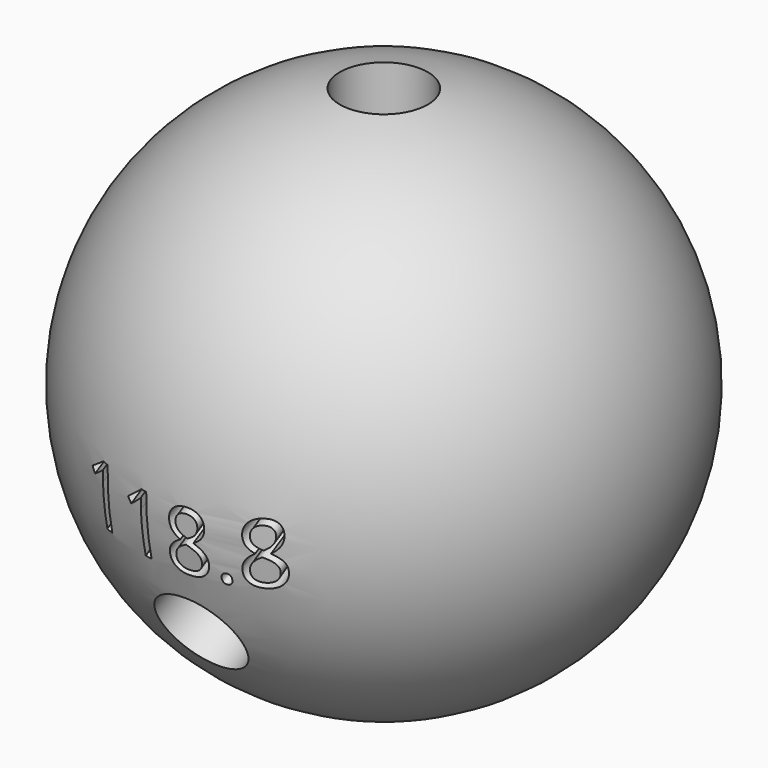
from build123d import *

# Parameters (mm, degrees)
F5_R          = 3.175
F6_DEPTH      = 76.2
F7_ANGLE      = 118.8
F8_ANGLE      = 119.3
F10_TEXT_SIZE = 5.7784387738
F11_DEPTH     = 6.35
F13_TEXT_SIZE = 6.645384969
F14_DEPTH     = 6.35


# Not quite as in the source:
# - Text() gives the source's letters only with a copy of the font that has no kerning and outlines rounded to 1/6400 em; it was checked with that copy


with BuildPart() as f2:
    # F0 (on Front) → F2 (revolve)
    with BuildSketch(Plane.XZ):
        with BuildLine():
            Line((0, -19.05), (0, 19.05))
            ThreePointArc((0, 19.05), (-19.05, 0), (0, -19.05))
        make_face()
    revolve(axis=Axis((0, 0, 0), (0, 0, 1)))

    # F10 (on offset) → F11 (cut)
    with BuildSketch(Plane(origin=(0, -17.8065517385, -9.7892346577), x_dir=(1, 0, 0), z_dir=(0, -0.87630668, -0.4817536741))):
        with Locations((-7.3158596642, 5.1700836048)):
            Text('118.8', F10_TEXT_SIZE, font='Open Sans', text_align=(TextAlign.LEFT, TextAlign.BOTTOM))
    extrude(amount=-F11_DEPTH, mode=Mode.SUBTRACT)

    # F13 (on offset) → F14 (cut)
    with BuildSketch(Plane(origin=(0, 17.2511046926, -10.7378669616), x_dir=(-1, 0, 0), z_dir=(0, 0.8489716876, -0.5284383347))):
        with Locations((-8.5034969068, 4.3885130435)):
            Text('119.3', F13_TEXT_SIZE, font='Open Sans', text_align=(TextAlign.LEFT, TextAlign.BOTTOM))
    extrude(amount=-F14_DEPTH, mode=Mode.SUBTRACT)


with BuildPart() as f6:
    # F5 (on offset) → F6 (new body)
    with BuildSketch(Plane.XY.offset(7.62)):
        Circle(F5_R)
    extrude(amount=F6_DEPTH)


with BuildPart() as f7_1:
    # F7: copy of F6
    add(f6.part.rotate(Axis((38.1614528596, 0, 0), (1, 0, 0)), F7_ANGLE))


with BuildPart() as f8_1:
    # F8: copy of F7_1
    add(f7_1.part.rotate(Axis((38.1614528596, 0, 0), (1, 0, 0)), F8_ANGLE))


with BuildPart() as f2_1:
    add(f2.part)

    # F15: cut F6, F8_1, F7_1
    add(f6.part, mode=Mode.SUBTRACT)
    add(f8_1.part, mode=Mode.SUBTRACT)
    add(f7_1.part, mode=Mode.SUBTRACT)


solid = f2_1.part
